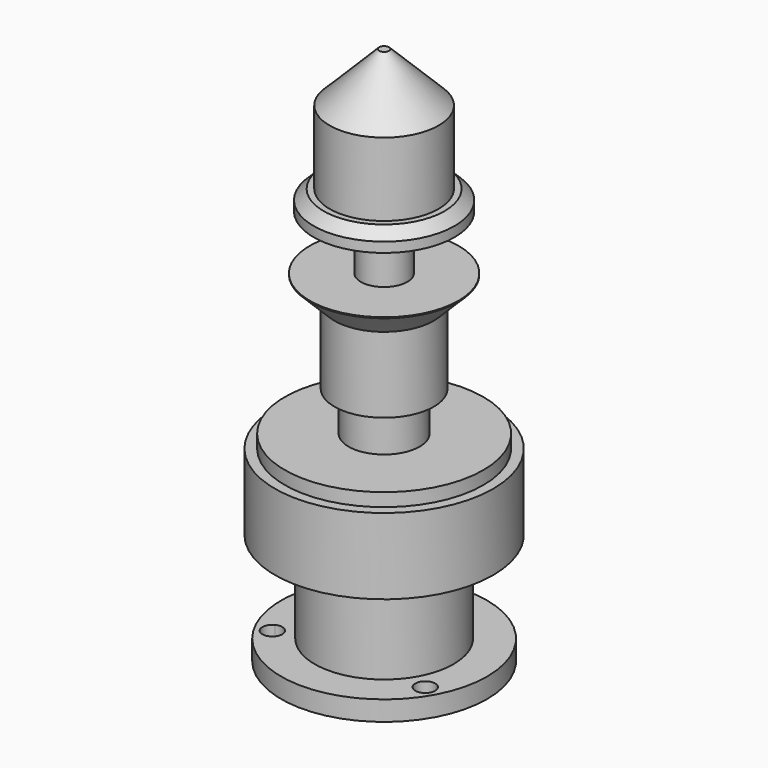
from build123d import *

# Parameters (mm, degrees)
F0_R      = 10.385
F1_DEPTH  = 2
F2_R      = 7
F3_DEPTH  = 9.2
F4_R      = 11
F4_R_2    = 7
F5_DEPTH  = 7.66
F6_R      = 10
F7_DEPTH  = 1.33
F8_R      = 3.585
F9_DEPTH  = 4
F10_R     = 5
F11_DEPTH = 7.62
F12_R     = 7.5
F13_DEPTH = 2.6
F14_SIZE  = 2.49999
F15_R     = 2.35
F16_DEPTH = 5.5
F17_R     = 7.1
F17_R_2   = 2.35
F18_DEPTH = 2
F19_SIZE  = 1
F20_R     = 5.5
F21_DEPTH = 12.4
F22_SIZE  = 5


# Not quite as in the source:
# - a fillet or chamfer is up to 0.001 mm smaller than in the source, because OpenCascade refuses the exact size


with BuildPart() as f1:
    # F0 (on Top) → F1 (new body)
    with BuildSketch(Plane.XY):
        Circle(F0_R)
        with BuildLine():
            ThreePointArc((0.9984206693, 8.8438202247), (6.6368646196, 5.9297578384), (8.9, 0))
            ThreePointArc((8.9, 0), (8.7125722812, -1.8168886165), (8.1581833158, -3.5572524491))
            ThreePointArc((8.1581833158, -3.5572524491), (8.5592590023, -3.9258612884), (8.7076260937, -4.45))
            ThreePointArc((8.7076260937, -4.45), (8.1830924715, -5.3297338936), (7.1597626465, -5.2865677756))
            ThreePointArc((7.1597626465, -5.2865677756), (0, -8.9), (-7.1597626465, -5.2865677756))
            ThreePointArc((-7.1597626465, -5.2865677756), (-8.5736514975, -4.95), (-8.1581833158, -3.5572524491))
            ThreePointArc((-8.1581833158, -3.5572524491), (-7.7076260937, 4.45), (-0.9984206693, 8.8438202247))
            ThreePointArc((-0.9984206693, 8.8438202247), (-0.028100985, 9.8996050893), (1, 8.9))
            ThreePointArc((1, 8.9), (0.9996050893, 8.871899015), (0.9984206693, 8.8438202247))
        make_face(mode=Mode.SUBTRACT)
        with BuildLine():
            ThreePointArc((8.1581833158, -3.5572524491), (8.7125722812, -1.8168886165), (8.9, 0))
            ThreePointArc((8.9, 0), (6.6368646196, 5.9297578384), (0.9984206693, 8.8438202247))
            ThreePointArc((0.9984206693, 8.8438202247), (0, 7.9), (-0.9984206693, 8.8438202247))
            ThreePointArc((-0.9984206693, 8.8438202247), (-7.7076260937, 4.45), (-8.1581833158, -3.5572524491))
            ThreePointArc((-8.1581833158, -3.5572524491), (-7.1834873821, -3.5983670914), (-6.7076260937, -4.45))
            ThreePointArc((-6.7076260937, -4.45), (-6.8278922, -4.9254663778), (-7.1597626465, -5.2865677756))
            ThreePointArc((-7.1597626465, -5.2865677756), (0, -8.9), (7.1597626465, -5.2865677756))
            ThreePointArc((7.1597626465, -5.2865677756), (6.8416006899, -3.95), (8.1581833158, -3.5572524491))
        make_face()
    extrude(amount=F1_DEPTH)

    # F2 (on face) → F3 (join)
    with BuildSketch(Plane.XY.offset(2)):
        Circle(F2_R)
    extrude(amount=F3_DEPTH)

    # F4 (on face) → F5 (join)
    with BuildSketch(Plane.XY.offset(11.2)):
        Circle(F4_R)
        Circle(F4_R_2, mode=Mode.SUBTRACT)
        Circle(F4_R_2)
    extrude(amount=F5_DEPTH)

    # F6 (on face) → F7 (join)
    with BuildSketch(Plane.XY.offset(18.86)):
        Circle(F6_R)
    extrude(amount=F7_DEPTH)

    # F8 (on face) → F9 (join)
    with BuildSketch(Plane.XY.offset(20.19)):
        Circle(F8_R)
    extrude(amount=F9_DEPTH)

    # F10 (on face) → F11 (join)
    with BuildSketch(Plane.XY.offset(24.19)):
        Circle(F10_R)
    extrude(amount=F11_DEPTH)

    # F12 (on face) → F13 (join)
    with BuildSketch(Plane.XY.offset(31.81)):
        Circle(F12_R)
    extrude(amount=F13_DEPTH)

    # F14 (size 2.5 in the source; OpenCascade refuses exactly that, so slightly less here)
    f14_edges = [f1.edges().sort_by_distance(p)[0] for p in [
        (-7.5, 0, 31.81),
    ]]
    chamfer(f14_edges, length=F14_SIZE)

    # F15 (on face) → F16 (join)
    with BuildSketch(Plane.XY.offset(34.41)):
        Circle(F15_R)
    extrude(amount=F16_DEPTH)


with BuildPart() as f18:
    # F17 (on face) → F18 (new body)
    with BuildSketch(Plane.XY.offset(39.91)):
        Circle(F17_R)
        Circle(F17_R_2, mode=Mode.SUBTRACT)
    extrude(amount=F18_DEPTH)

    # F19
    f19_edges = [f18.edges().sort_by_distance(p)[0] for p in [
        (-7.1, 0, 41.91),
    ]]
    chamfer(f19_edges, length=F19_SIZE)

    # F20 (on face) → F21 (join)
    with BuildSketch(Plane.XY.offset(41.91)):
        Circle(F20_R)
    extrude(amount=F21_DEPTH)

    # F22
    f22_edges = [f18.edges().sort_by_distance(p)[0] for p in [
        (-5.5, 0, 54.31),
    ]]
    chamfer(f22_edges, length=F22_SIZE)


solid = Compound([f1.part, f18.part])
